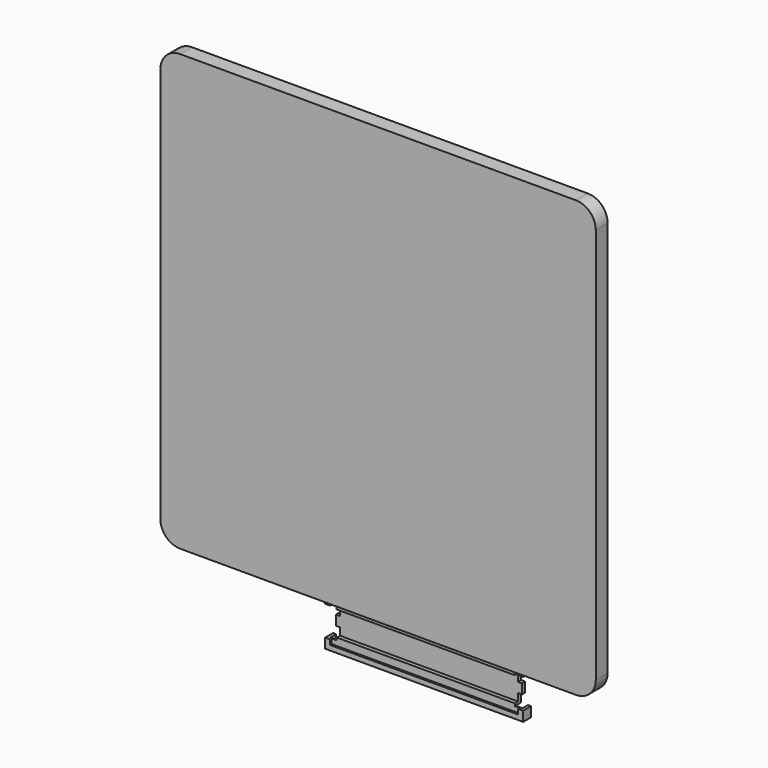
from build123d import *

# Parameters (mm, degrees)
F0_R     = 5
F1_DEPTH = 7.5
F2_W     = 80
F2_H     = 2.5
F3_DEPTH = 5
F4_W     = 94
F4_H     = 12.5
F5_DEPTH = 3
F6_W     = 97
F6_H     = 3.5
F7_DEPTH = 5
F8_W     = 95
F8_H     = 20
F9_DEPTH = 1


with BuildPart() as f1:
    # F0 (on Front) → F1 (new body)
    with BuildSketch(Plane.XZ):
        with BuildLine():
            Line((33.4357412159, 189.6795940399), (-166.5642587841, 189.6795940399))
            ThreePointArc((-166.5642587841, 189.6795940399), (-173.6353265959, 186.7506618518), (-176.5642587841, 179.6795940399))
            Line((-176.5642587841, 179.6795940399), (-176.5642587841, -20.3204059601))
            ThreePointArc((-176.5642587841, -20.3204059601), (-173.6353265959, -27.3914737719), (-166.5642587841, -30.3204059601))
            Line((-166.5642587841, -30.3204059601), (33.4357412159, -30.3204059601))
            ThreePointArc((33.4357412159, -30.3204059601), (40.5068090278, -27.3914737719), (43.4357412159, -20.3204059601))
            Line((43.4357412159, -20.3204059601), (43.4357412159, 179.6795940399))
            ThreePointArc((43.4357412159, 179.6795940399), (40.5068090278, 186.7506618518), (33.4357412159, 189.6795940399))
        make_face()
        with Locations((-116.5642587841, 29.6795940399)):
            Circle(F0_R, mode=Mode.SUBTRACT)
        with Locations((-16.5642587841, 29.6795940399)):
            Circle(F0_R, mode=Mode.SUBTRACT)
        with Locations((-116.5642587841, 129.6795940399)):
            Circle(F0_R, mode=Mode.SUBTRACT)
        with Locations((-16.5642587841, 129.6795940399)):
            Circle(F0_R, mode=Mode.SUBTRACT)
        with Locations((-116.5642587841, 129.6795940399)):
            Circle(F0_R)
        with Locations((-16.5642587841, 129.6795940399)):
            Circle(F0_R)
        with Locations((-16.5642587841, 29.6795940399)):
            Circle(F0_R)
        with Locations((-116.5642587841, 29.6795940399)):
            Circle(F0_R)
    extrude(amount=F1_DEPTH)


with BuildPart() as f3:
    # F2 (on Front) → F3 (new body)
    with BuildSketch(Plane.XZ):
        Polygon((-95.2747841366, -52.6743675989), (-90.2747841366, -52.6743675989), (4.7252158634, -52.6743675989), (4.7252158634, -47.6743675989), (-0.2747841366, -47.6743675989), (-0.2747841366, -42.6743675989), (1.7252158634, -42.6743675989), (1.7252158634, -37.6743675989), (-0.2747841366, -37.6743675989), (-0.2747841366, -32.6743675989), (4.7252158634, -32.6743675989), (4.7252158634, -27.6743675989), (-90.2747841366, -27.6743675989), (-95.2747841366, -27.6743675989), (-95.2747841366, -32.6743675989), (-90.2747841366, -32.6743675989), (-90.2747841366, -37.6743675989), (-92.2747841366, -37.6743675989), (-92.2747841366, -42.6743675989), (-90.2747841366, -42.6743675989), (-90.2747841366, -47.6743675989), (-95.2747841366, -47.6743675989), align=None)
        with Locations((-45.2747841366, -31.4243675989)):
            Rectangle(F2_W, F2_H, mode=Mode.SUBTRACT)
    extrude(amount=F3_DEPTH)

    # F4 (on face) → F5 (cut)
    with BuildSketch(Plane.XZ.offset(5)):
        with Locations((-45.2747841366, -40.1743675989)):
            Rectangle(F4_W, F4_H)
    extrude(amount=-F5_DEPTH, mode=Mode.SUBTRACT)

    # F6 (on face) → F7 (cut)
    with BuildSketch(Plane(origin=(0, 0, -52.6743675989), x_dir=(1, 0, 0), z_dir=(0, 0, -1))):
        with Locations((-45.2747841366, 1.75)):
            Rectangle(F6_W, F6_H)
    extrude(amount=-F7_DEPTH, mode=Mode.SUBTRACT)

    # F8 (on face) → F9 (cut)
    with BuildSketch(Plane.XZ.offset(5)):
        with Locations((-45.2747841366, -40.1743675989)):
            Rectangle(F8_W, F8_H)
    extrude(amount=-F9_DEPTH, mode=Mode.SUBTRACT)


solid = Compound([f1.part, f3.part])
